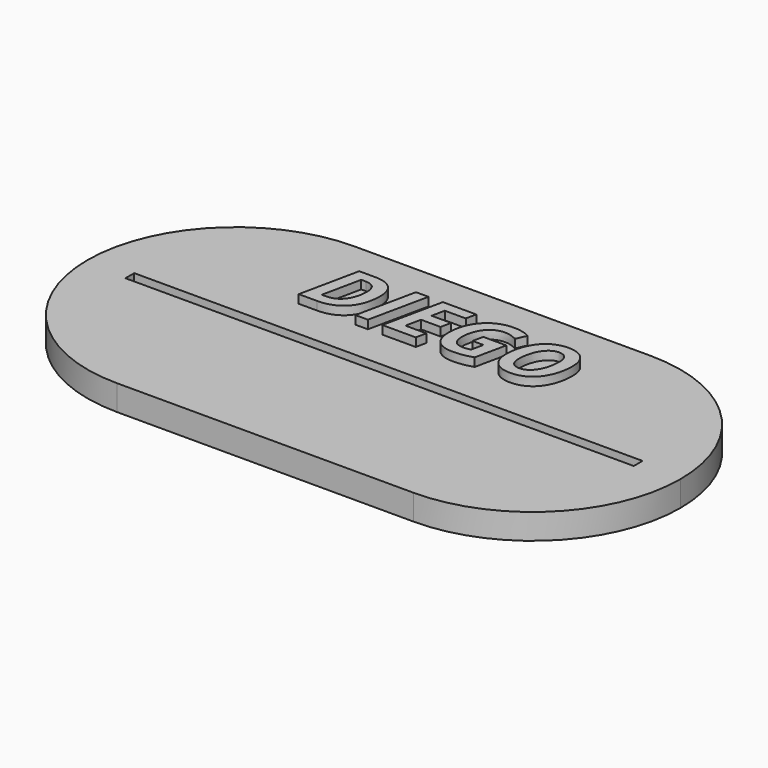
from build123d import *

# Parameters (mm, degrees)
F0_W         = 70
F0_H         = 35
F0_W_2       = 60
F0_H_2       = 1.3
F1_DEPTH     = 3
F2_R         = 17.49999
F3_SIZE      = 1
F4_TEXT_SIZE = 9.8863564846
F5_DEPTH     = 1


# Not quite as in the source:
# - a fillet or chamfer is up to 0.001 mm smaller than in the source, because OpenCascade refuses the exact size
# - Text() gives the source's letters only with a copy of the font that has no kerning and outlines rounded to 1/6400 em; it was checked with that copy


with BuildPart() as f1:
    # F0 (on Top) → F1 (new body)
    with BuildSketch(Plane.XY):
        with Locations((35, 17.5)):
            Rectangle(F0_W, F0_H)
        with Locations((35, 17.5)):
            Rectangle(F0_W_2, F0_H_2, mode=Mode.SUBTRACT)
    extrude(amount=F1_DEPTH)

    # F2 (radius 17.5 in the source; OpenCascade refuses exactly that, so slightly less here)
    f2_edges = [f1.edges().sort_by_distance(p)[0] for p in [
        (70, 0, 1.5),
        (70, 35, 1.5),
        (0, 35, 1.5),
        (0, 0, 1.5),
    ]]
    fillet(f2_edges, radius=F2_R)

    # F3
    f3_edges = [f1.edges().sort_by_distance(p)[0] for p in [
        (35, 16.85, 0),
        (35, 18.15, 0),
    ]]
    chamfer(f3_edges, length=F3_SIZE)


with BuildPart() as f5:
    # F4 (on face) → F5 (new body)
    with BuildSketch(Plane.XY.offset(3)):
        with Locations((20.4017814249, 22.8461325169)):
            Text('DIEGO', F4_TEXT_SIZE, font='Open Sans', font_style=FontStyle.BOLDITALIC, text_align=(TextAlign.LEFT, TextAlign.BOTTOM))
    extrude(amount=F5_DEPTH)


solid = Compound([f1.part, f5.part])
